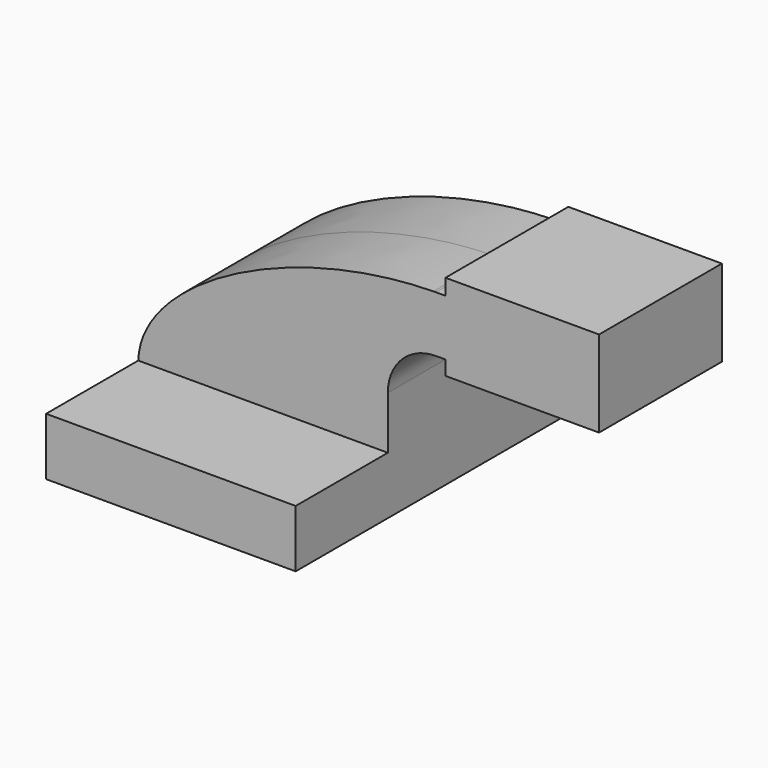
from build123d import *

# Parameters (mm, degrees)
F1_DEPTH = 63.5
F2_DEPTH = 25.4
F0_W     = 25.4
F0_H     = 18.5420008242
F0_H_2   = 5.2577991758
F0_H_3   = 4.7752
F3_DEPTH = 25.4


with BuildPart() as f1:
    # F0 (on Front) → F1 (new body, symmetric)
    with BuildSketch(Plane.XZ):
        Polygon((-41.275, 9.525), (-41.275, -9.525), (41.275, -9.525), (41.275, 9.525), (22.7329991758, 9.525), align=None)
    extrude(amount=F1_DEPTH, both=True)

    # F0 (on Front) → F2 (join, symmetric)
    with BuildSketch(Plane.XZ):
        with BuildLine():
            Line((22.7329991758, 9.525), (41.275, 9.525))
            Line((41.275, 9.525), (41.275, 27.0002))
            ThreePointArc((41.275, 27.0002), (45.9246798487, 38.2255201513), (57.15, 42.8752))
            Line((57.15, 42.8752), (60.325, 42.8752))
            Line((60.325, 42.8752), (60.325, 61.4172008242))
            Line((60.325, 61.4172008242), (57.15, 61.4172008242))
            add(Edge.make_bspline(
                [(56.3787146856, 61.4085574833), (56.6358462416, 61.412165765), (56.8929439024, 61.4150481962), (57.15, 61.4172008242)],
                knots=[110.67146519, 110.67146519, 110.67146519, 110.67146519, 111.2667116948, 111.2667116948, 111.2667116948, 111.2667116948], degree=3))
            ThreePointArc((56.3787146856, 61.4085574833), (32.5423256581, 51.0624590215), (22.7329991758, 27.0002))
            Line((22.7329991758, 27.0002), (22.7329991758, 9.525))
        make_face()
    extrude(amount=F2_DEPTH, both=True)

    # F0 (on Front) → F3 (join, symmetric)
    with BuildSketch(Plane.XZ):
        Polygon((-41.275, 9.525), (-41.275, -9.525), (41.275, -9.525), (41.275, 9.525), (22.7329991758, 9.525), align=None)
        with BuildLine():
            add(Edge.make_bspline(
                [(-41.275, 9.525), (-40.4075770381, 34.9754176722), (8.5714183415, 60.7376861335), (56.3787146856, 61.4085574833)],
                knots=[0, 0, 0, 0, 110.67146519, 110.67146519, 110.67146519, 110.67146519], degree=3))
            Line((-41.275, 9.525), (22.7329991758, 9.525))
            Line((22.7329991758, 9.525), (22.7329991758, 27.0002))
            ThreePointArc((22.7329991758, 27.0002), (32.5423256581, 51.0624590215), (56.3787146856, 61.4085574833))
        make_face()
        with BuildLine():
            Line((22.7329991758, 9.525), (41.275, 9.525))
            Line((41.275, 9.525), (41.275, 27.0002))
            ThreePointArc((41.275, 27.0002), (45.9246798487, 38.2255201513), (57.15, 42.8752))
            Line((57.15, 42.8752), (60.325, 42.8752))
            Line((60.325, 42.8752), (60.325, 61.4172008242))
            Line((60.325, 61.4172008242), (57.15, 61.4172008242))
            add(Edge.make_bspline(
                [(56.3787146856, 61.4085574833), (56.6358462416, 61.412165765), (56.8929439024, 61.4150481962), (57.15, 61.4172008242)],
                knots=[110.67146519, 110.67146519, 110.67146519, 110.67146519, 111.2667116948, 111.2667116948, 111.2667116948, 111.2667116948], degree=3))
            ThreePointArc((56.3787146856, 61.4085574833), (32.5423256581, 51.0624590215), (22.7329991758, 27.0002))
            Line((22.7329991758, 27.0002), (22.7329991758, 9.525))
        make_face()
        with Locations((73.025, 52.1462004121)):
            Rectangle(F0_W, F0_H)
        with Locations((73.025, 64.0461004121)):
            Rectangle(F0_W, F0_H_2)
        with Locations((73.025, 40.4876)):
            Rectangle(F0_W, F0_H_3)
        Polygon((85.725, 66.675), (85.725, 61.4172008242), (85.725, 42.8752), (85.725, 38.1), (111.125, 38.1), (111.125, 66.675), align=None)
    extrude(amount=F3_DEPTH, both=True)


solid = f1.part
